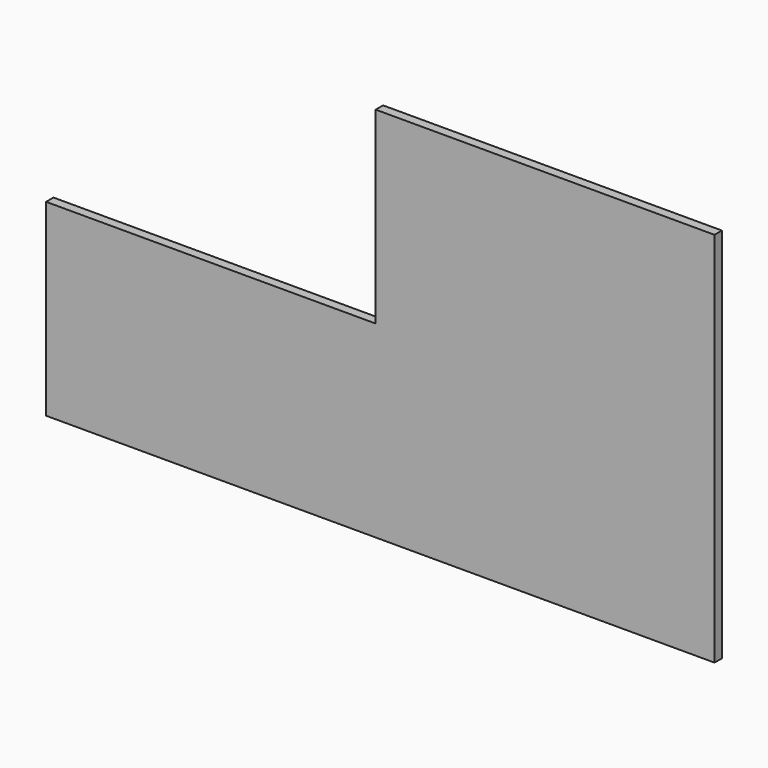
from build123d import *

# Parameters (mm, degrees)
F1_DEPTH = 10


# Not quite as in the source:
# - a feature names something its author has since deleted; it is built from what else it names


with BuildPart() as f1:
    # F0 (on Front) → F1 (new body)
    with BuildSketch(Plane.XZ):
        Polygon((256.5041949631, 441.1109750425), (256.5041949631, 237.9109750425), (977.7117949631, 237.9109750425), (977.7117949631, 644.3109750425), (612.1041949631, 644.3109750425), (612.1041949631, 441.1109750425), align=None)
    extrude(amount=F1_DEPTH)


solid = f1.part
